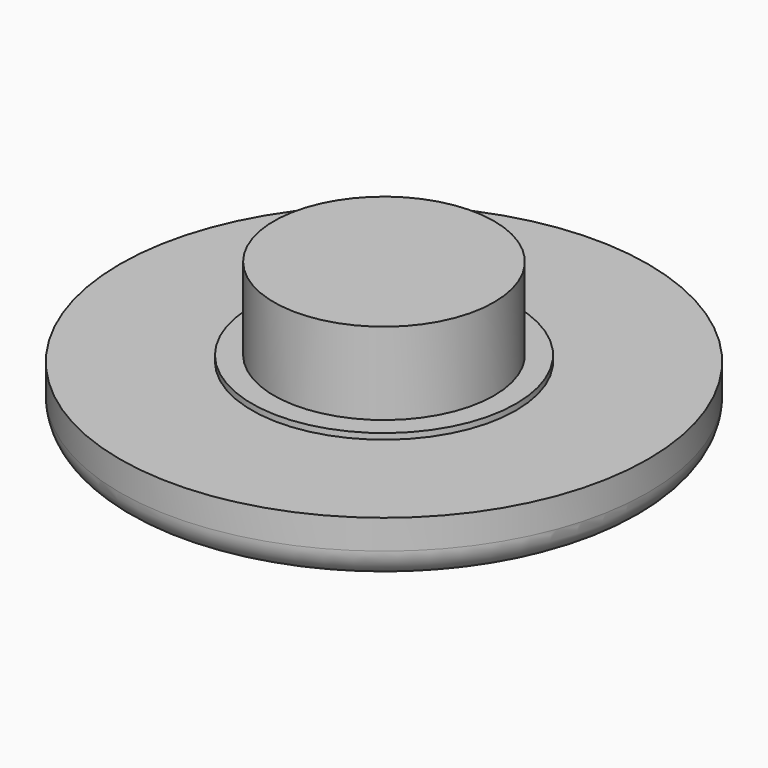
from build123d import *

# Parameters (mm, degrees)
F0_R         = 9
F1_DEPTH     = 2
F2_R         = 3.75
F3_DEPTH     = 3
F4_R         = 1
F5_TEXT_SIZE = 17.4729013462
F6_DEPTH     = 1.5
F7_R         = 4.5
F7_R_2       = 3.75
F8_DEPTH     = 0.2


# Not quite as in the source:
# - Text() gives the source's letters only with a copy of the font that has no kerning and outlines rounded to 1/6400 em; it was checked with that copy


with BuildPart() as f1:
    # F0 (on Top) → F1 (new body)
    with BuildSketch(Plane.XY):
        Circle(F0_R)
    extrude(amount=F1_DEPTH)

    # F2 (on face) → F3 (join)
    with BuildSketch(Plane.XY.offset(2)):
        Circle(F2_R)
    extrude(amount=F3_DEPTH)

    # F4
    f4_edges = [f1.edges().sort_by_distance(p)[0] for p in [
        (-9, 0, 0),
    ]]
    fillet(f4_edges, radius=F4_R)

    # F5 (on face) → F6 (cut)
    with BuildSketch(Plane(origin=(0, 0, 0), x_dir=(1, 0, 0), z_dir=(0, 0, -1))):
        with Locations((-4.9278698813, -6.2784180054)):
            Text('S', F5_TEXT_SIZE, font='Open Sans', text_align=(TextAlign.LEFT, TextAlign.BOTTOM))
    extrude(amount=-F6_DEPTH, mode=Mode.SUBTRACT)

    # F7 (on face) → F8 (join)
    with BuildSketch(Plane.XY.offset(2)):
        Circle(F7_R)
        Circle(F7_R_2, mode=Mode.SUBTRACT)
    extrude(amount=F8_DEPTH)


solid = f1.part
